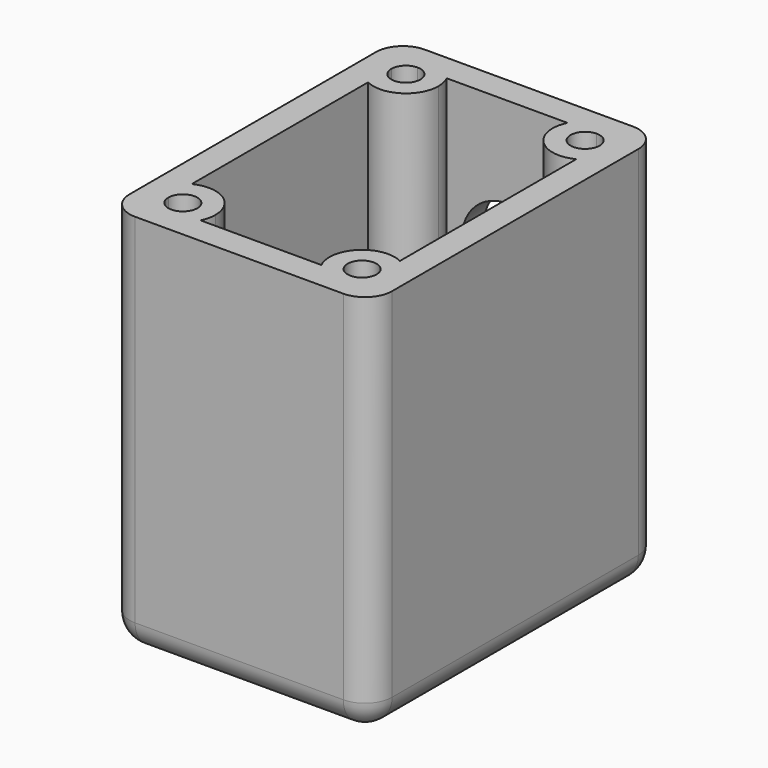
from build123d import *

# Parameters (mm, degrees)
F0_W      = 29
F0_H      = 40
F0_W_2    = 15
F0_H_2    = 19
F1_DEPTH  = 2.5
F2_W      = 29
F2_H      = 40
F2_W_2    = 23
F2_H_2    = 34
F3_DEPTH  = 40
F5_DEPTH  = 40
F6_R      = 1.6
F7_DEPTH  = 25
F8_R      = 2.99999
F9_R      = 5
F10_DEPTH = 3


# Not quite as in the source:
# - a fillet or chamfer is up to 0.001 mm smaller than in the source, because OpenCascade refuses the exact size


with BuildPart() as f1:
    # F0 (on Top) → F1 (new body)
    with BuildSketch(Plane.XY):
        Rectangle(F0_W, F0_H)
        Rectangle(F0_W_2, F0_H_2, mode=Mode.SUBTRACT)
    extrude(amount=F1_DEPTH)

    # F2 (on face) → F3 (join)
    with BuildSketch(Plane.XY.offset(2.5)):
        Rectangle(F2_W, F2_H)
        Rectangle(F2_W_2, F2_H_2, mode=Mode.SUBTRACT)
    extrude(amount=F3_DEPTH)

    # F4 (on face) → F5 (join, through all)
    with BuildSketch(Plane.XY.offset(2.5)):
        with BuildLine():
            ThreePointArc((-11.5, 12.175097), (-8.002633, 12.340588), (-6.3, 15.4))
            ThreePointArc((-6.3, 15.4), (-6.395028, 16.22169), (-6.675097, 17))
            Line((-6.675097, 17), (-9.9, 17))
            ThreePointArc((-9.9, 17), (-8.768629, 16.531371), (-8.3, 15.4))
            ThreePointArc((-8.3, 15.4), (-9.9, 13.8), (-11.5, 15.4))
            Line((-11.5, 15.4), (-11.5, 12.175097))
        make_face()
        with BuildLine():
            ThreePointArc((-11.5, 15.4), (-11.031371, 16.531371), (-9.9, 17))
            Line((-9.9, 17), (-11.5, 17))
            Line((-11.5, 17), (-11.5, 15.4))
        make_face()
        with BuildLine():
            Line((9.9, 17), (6.675097, 17))
            ThreePointArc((6.675097, 17), (7.354416, 12.854416), (11.5, 12.175097))
            Line((11.5, 12.175097), (11.5, 15.4))
            ThreePointArc((11.5, 15.4), (8.768629, 14.268629), (9.9, 17))
        make_face()
        with BuildLine():
            Line((11.5, 17), (9.9, 17))
            ThreePointArc((9.9, 17), (11.031371, 16.531371), (11.5, 15.4))
            Line((11.5, 15.4), (11.5, 17))
        make_face()
        with BuildLine():
            ThreePointArc((-9.9, -17), (-11.031371, -16.531371), (-11.5, -15.4))
            Line((-11.5, -15.4), (-11.5, -17))
            Line((-11.5, -17), (-9.9, -17))
        make_face()
        with BuildLine():
            ThreePointArc((-6.3, -15.4), (-8.002633, -12.340588), (-11.5, -12.175097))
            Line((-11.5, -12.175097), (-11.5, -15.4))
            ThreePointArc((-11.5, -15.4), (-9.9, -13.8), (-8.3, -15.4))
            ThreePointArc((-8.3, -15.4), (-8.768629, -16.531371), (-9.9, -17))
            Line((-9.9, -17), (-6.675097, -17))
            ThreePointArc((-6.675097, -17), (-6.395028, -16.22169), (-6.3, -15.4))
        make_face()
        with BuildLine():
            Line((11.5, -15.4), (11.5, -12.175097))
            ThreePointArc((11.5, -12.175097), (7.354416, -12.854416), (6.675097, -17))
            Line((6.675097, -17), (9.9, -17))
            ThreePointArc((9.9, -17), (8.768629, -14.268629), (11.5, -15.4))
        make_face()
        with BuildLine():
            Line((11.5, -17), (11.5, -15.4))
            ThreePointArc((11.5, -15.4), (11.031371, -16.531371), (9.9, -17))
            Line((9.9, -17), (11.5, -17))
        make_face()
    extrude(amount=F5_DEPTH)

    # F6 (on face) → F7 (cut)
    with BuildSketch(Plane(origin=(0, 0, 0), x_dir=(1, 0, 0), z_dir=(0, 0, -1))):
        with Locations((-9.9, 15.4)):
            Circle(F6_R)
        with Locations((9.9, 15.4)):
            Circle(F6_R)
        with Locations((9.9, -15.4)):
            Circle(F6_R)
        with Locations((-9.9, -15.4)):
            Circle(F6_R)
    extrude(amount=-F7_DEPTH, mode=Mode.SUBTRACT)

    # F8 (radius 3 in the source; OpenCascade refuses exactly that, so slightly less here)
    f8_edges = [f1.edges().sort_by_distance(p)[0] for p in [
        (-14.5, -20, 21.25),
        (14.5, -20, 21.25),
        (-14.5, 20, 21.25),
        (14.5, 20, 21.25),
        (-14.5, 0, 0),
        (0, 20, 0),
        (14.5, 0, 0),
        (0, -20, 0),
    ]]
    fillet(f8_edges, radius=F8_R)

    # F9 (on face) → F10 (cut, through all)
    with BuildSketch(Plane.XZ.offset(-17)):
        with Locations((0, 27.5)):
            Circle(F9_R)
    extrude(amount=-F10_DEPTH, mode=Mode.SUBTRACT)


solid = f1.part
